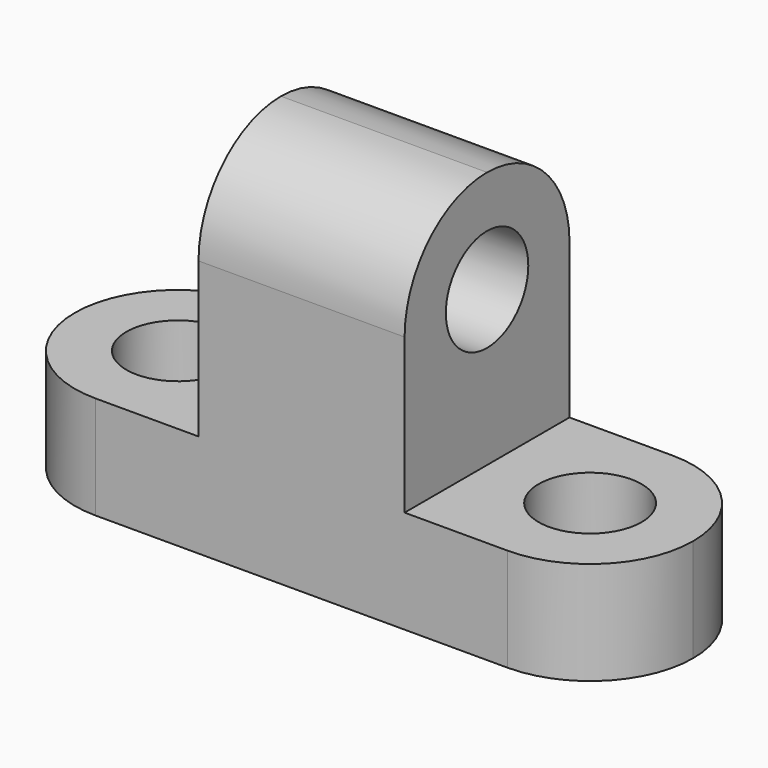
from build123d import *

# Parameters (mm, degrees)
F1_DEPTH = 25.4
F2_R     = 6.35
F3_DEPTH = 76.2
F4_R     = 6.35
F5_DEPTH = 12.7


# Not quite as in the source:
# - a feature names something its author has since deleted; it is built from what else it names


with BuildPart() as f1:
    # F0 (on Front) → F1 (new body)
    with BuildSketch(Plane.XZ):
        Polygon((0, 12.7), (0, 0), (76.2, 0), (76.2, 12.7), (50.8, 12.7), (50.8, 44.45), (25.4, 44.45), (25.4, 12.7), align=None)
    extrude(amount=F1_DEPTH)

    # F2 (on Right) → F3 (cut)
    with BuildSketch(Plane.YZ):
        with Locations((-12.7, 31.75)):
            Circle(F2_R)
        with BuildLine():
            ThreePointArc((-25.4, 31.75), (-21.6802561211, 40.7302561211), (-12.7, 44.45))
            Line((-12.7, 44.45), (-25.4, 44.45))
            Line((-25.4, 44.45), (-25.4, 31.75))
        make_face()
        with BuildLine():
            ThreePointArc((-12.7, 44.45), (-3.7197438789, 40.7302561211), (0, 31.75))
            Line((0, 31.75), (0, 44.45))
            Line((0, 44.45), (-12.7, 44.45))
        make_face()
    extrude(amount=F3_DEPTH, mode=Mode.SUBTRACT)

    # F4 (on Top) → F5 (cut)
    with BuildSketch(Plane.XY):
        with Locations((63.5, -12.7)):
            Circle(F4_R)
        with BuildLine():
            ThreePointArc((12.7, -25.4), (3.7197438789, -21.6802561211), (0, -12.7))
            Line((0, -12.7), (0, -25.4))
            Line((0, -25.4), (12.7, -25.4))
        make_face()
        with BuildLine():
            ThreePointArc((0, -12.7), (3.7197438789, -3.7197438789), (12.7, 0))
            Line((12.7, 0), (0, 0))
            Line((0, 0), (0, -12.7))
        make_face()
        with Locations((12.7, -12.7)):
            Circle(F4_R)
        with BuildLine():
            ThreePointArc((76.2, -12.7), (72.4802561211, -21.6802561211), (63.5, -25.4))
            Line((63.5, -25.4), (76.2, -25.4))
            Line((76.2, -25.4), (76.2, -12.7))
        make_face()
        with BuildLine():
            ThreePointArc((63.5, 0), (72.4802561211, -3.7197438789), (76.2, -12.7))
            Line((76.2, -12.7), (76.2, 0))
            Line((76.2, 0), (63.5, 0))
        make_face()
    extrude(amount=F5_DEPTH, mode=Mode.SUBTRACT)


solid = f1.part
